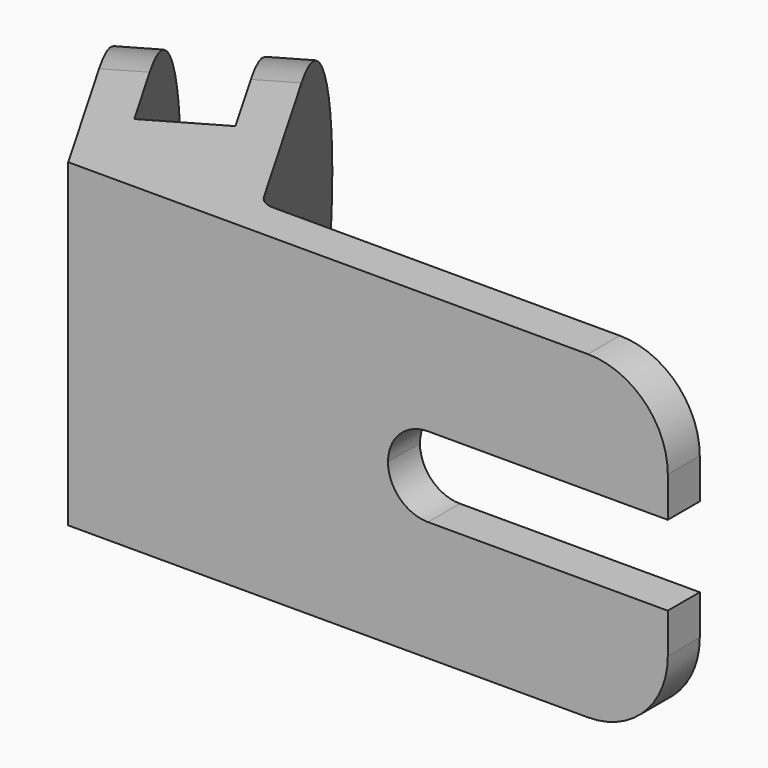
from build123d import *

# Parameters (mm, degrees)
F1_DEPTH      = 40
F1_DEPTH_BACK = 40
F2_R          = 5
F3_R          = 39.99999
F4_R          = 10
F5_DEPTH      = 52.2
F7_DEPTH      = 25
F8_R          = 20


# Not quite as in the source:
# - a fillet or chamfer is up to 0.001 mm smaller than in the source, because OpenCascade refuses the exact size


with BuildPart() as f1:
    # F0 (on Top) → F1 (new body, two sides)
    with BuildSketch(Plane.XY) as f1_sk:
        Polygon((-44.4148934171, 0), (105.5851065829, 0), (105.5851065829, 10), (-4.0003745738, 10), (-49.7738772657, 89.2820323028), (-58.4341313035, 84.2820323028), (-28.4341313035, 32.3205080757), (-45.7546393792, 22.3205080757), (-75.7546393792, 74.2820323028), (-84.4148934171, 69.2820323028), align=None)
    extrude(amount=F1_DEPTH)
    extrude(f1_sk.sketch, amount=-F1_DEPTH_BACK)

    # F2
    f2_edges = [f1.edges().sort_by_distance(p)[0] for p in [
        (-4.000375, 10, 0),
    ]]
    fillet(f2_edges, radius=F2_R)

    # F3 (radius 40 in the source; OpenCascade refuses exactly that, so slightly less here)
    f3_edges = [f1.edges().sort_by_distance(p)[0] for p in [
        (-54.104004, 86.782032, 40),
        (-80.084766, 71.782032, 40),
        (-80.084766, 71.782032, -40),
        (-54.104004, 86.782032, -40),
    ]]
    fillet(f3_edges, radius=F3_R)

    # F4 (on face) → F5 (cut)
    with BuildSketch(Plane(origin=(1.3298460886, 0.7677869972, 0), x_dir=(-0.5, 0.8660254038, 0), z_dir=(0.8660254038, 0.5, 0))):
        with Locations((60.2471926707, 0)):
            Circle(F4_R)
    extrude(amount=-F5_DEPTH, mode=Mode.SUBTRACT)

    # F6 (on face) → F7 (cut)
    with BuildSketch(Plane(origin=(0, 10, 0), x_dir=(-1, 0, 0), z_dir=(0, 1, 0))):
        with BuildLine():
            ThreePointArc((-45.5851065829, -10), (-55.5851065829, 0), (-45.5851065829, 10))
            Line((-45.5851065829, 10), (-105.5851065829, 10))
            Line((-105.5851065829, 10), (-105.5851065829, -10))
            Line((-105.5851065829, -10), (-45.5851065829, -10))
        make_face()
        with BuildLine():
            ThreePointArc((-45.5851065829, -10), (-38.5140387711, -7.0710678119), (-35.5851065829, 0))
            ThreePointArc((-35.5851065829, 0), (-38.5140387711, 7.0710678119), (-45.5851065829, 10))
            ThreePointArc((-45.5851065829, 10), (-55.5851065829, 0), (-45.5851065829, -10))
        make_face()
    extrude(amount=-F7_DEPTH, mode=Mode.SUBTRACT)

    # F8
    f8_edges = [f1.edges().sort_by_distance(p)[0] for p in [
        (105.585107, 5, -40),
        (105.585107, 5, 40),
    ]]
    fillet(f8_edges, radius=F8_R)


solid = f1.part
